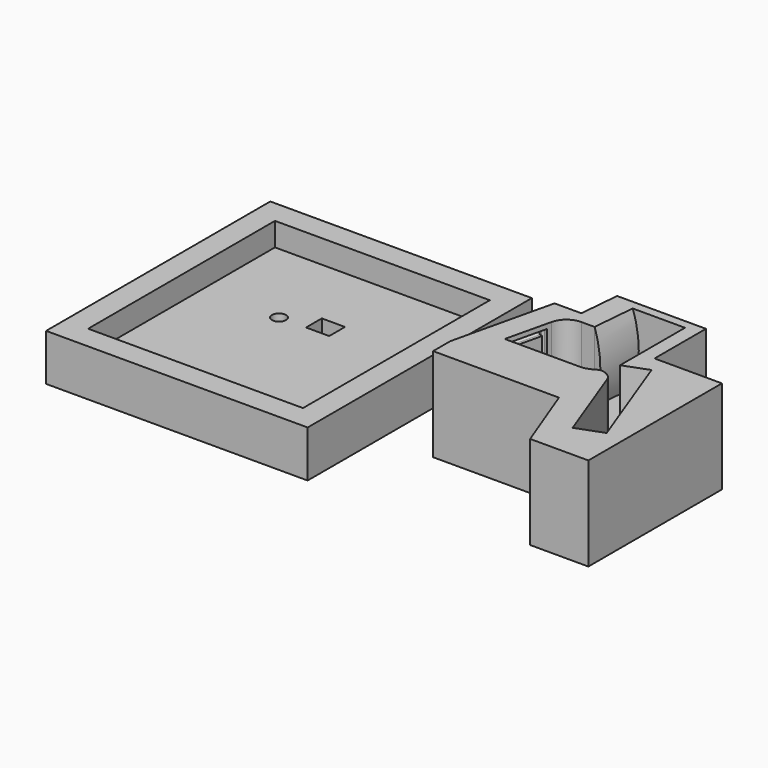
from build123d import *

# Parameters (mm, degrees)
F1_DEPTH      = 15
F4_DEPTH      = 9.2
F4_DEPTH_BACK = 1
F6_R          = 1.5
F7_DEPTH      = 20
F9_R          = 1.5
F10_DEPTH     = 5
F11_W         = 56
F11_H         = 60
F11_R         = 1.5
F11_W_2       = 4.962
F11_H_2       = 4.2207975686
F12_DEPTH     = 5
F14_W         = 56
F14_H         = 60
F14_W_2       = 46
F14_H_2       = 50
F15_DEPTH     = 5
F20_W         = 7.9759681362
F20_H         = 13
F20_W_2       = 5.9759681362
F20_H_2       = 11
F21_DEPTH     = 1
F22_R         = 0.4


# Not quite as in the source:
# - the program builds the solid bodies; features that only make, move or delete a surface that nothing else refers to are left out


with BuildPart() as f1:
    # F0 (on Top) → F1 (new body)
    with BuildSketch(Plane.XY):
        with BuildLine():
            Line((2.2764293651, 9.7127652912), (0, 0))
            Line((0, 0), (16, 0))
            ThreePointArc((16, 0), (17.4448615439, 0.2133127198), (18.7664401496, 0.8350499525))
            ThreePointArc((18.7664401496, 0.8350499525), (19.8489592754, 1.1689252442), (20.9391965895, 0.8611867726))
            ThreePointArc((20.9391965895, 0.8611867726), (21.8699515292, 0.2737220948), (22.4677167157, -0.6504512046))
            Line((22.4677167157, -0.6504512046), (28.953752481, -18.0237612902))
            Line((28.953752481, -18.0237612902), (34.5748015694, -15.9252362972))
            Line((34.5748015694, -15.9252362972), (26.1807015974, 6.5589600562))
            Line((26.1807015974, 6.5589600562), (21, 4.6248314599))
            Line((21, 4.6248314599), (21, 22))
            Line((21, 22), (9.8, 22))
            Line((9.8, 22), (9.0007942351, 12.8091337038))
            ThreePointArc((9.0007942351, 12.8091337038), (8.9975896779, 12.8026290109), (8.9908318292, 12.8))
            Line((8.9908318292, 12.8), (6.1708946074, 12.8))
            ThreePointArc((6.1708946074, 12.8), (3.6860466407, 11.9345702389), (2.2764293651, 9.7127652912))
        make_face()
    extrude(amount=F1_DEPTH)

    # F3 (on face) → F4 (cut, two sides)
    with BuildSketch(Plane(origin=(1.9722326454, 22.6806754221, 0), x_dir=(0.9962405882, -0.0866296164, 0), z_dir=(-0.0866296164, -0.9962405882, 0))) as f4_sk:
        with BuildLine():
            Line((7.8573062043, 15), (7.8573062043, 0))
            ThreePointArc((7.8573062043, 0), (9.161162664, 7.5), (7.8573062043, 15))
        make_face()
    extrude(amount=F4_DEPTH, mode=Mode.SUBTRACT)
    extrude(f4_sk.sketch, amount=-F4_DEPTH_BACK, mode=Mode.SUBTRACT)


with BuildPart() as f7:
    # F6 (on offset) → F7 (new body)
    with BuildSketch(Plane.XY.offset(-5)):
        Polygon((23.9650979638, 23.9009789079), (4.9464345222, 23.9009789079), (4.1964484146, 15.2761386707), (-1.5551482583, 15.2761386707), (-6.6067720969, -6.2774563741), (-6.6067720969, -10.9053393826), (20.3434042633, -10.9053393826), (25.9253627227, -25.5990210921), (38.3932279031, -25.5990210921), (38.3932279031, 10.140940547), (23.9650979638, 10.140940547), align=None)
        with Locations((16, 5)):
            Circle(F6_R, mode=Mode.SUBTRACT)
    extrude(amount=F7_DEPTH)

    # F8: cut F1
    add(f1.part, mode=Mode.SUBTRACT)

    # F9 (on offset) → F10 (cut)
    with BuildSketch(Plane.XY.offset(-5)):
        with Locations((16, 5)):
            Circle(F9_R)
    extrude(amount=F10_DEPTH, mode=Mode.SUBTRACT)

    # F20 (on offset) → F21 (cut)
    with BuildSketch(Plane(origin=(0, 0, 0), x_dir=(0.2281913228, 0.9736163106, 0), z_dir=(0.9736163106, -0.2281913228, 0))):
        with Locations((4.9879840681, 7.5)):
            Rectangle(F20_W, F20_H)
        with Locations((4.9879840681, 7.5)):
            Rectangle(F20_W_2, F20_H_2, mode=Mode.SUBTRACT)
    extrude(amount=-F21_DEPTH, mode=Mode.SUBTRACT)

    # F22
    f22_edges = [f7.edges().sort_by_distance(p)[0] for p in [
        (1.074622, 8.96734, 7.5),
        (0.164598, 5.084574, 14),
        (-0.745425, 1.201808, 7.5),
        (0.164598, 5.084574, 1),
        (0.84643, 7.993724, 7.5),
        (0.164598, 5.084574, 13),
        (-0.517234, 2.175424, 7.5),
        (0.164598, 5.084574, 2),
    ]]
    fillet(f22_edges, radius=F22_R)


with BuildPart() as f12:
    # F11 (on offset) → F12 (new body)
    with BuildSketch(Plane.XY.offset(-5)):
        with Locations((-45.7067461014, -0.5990204215)):
            Rectangle(F11_W, F11_H)
        with Locations((-52.3137461014, 5)):
            Circle(F11_R, mode=Mode.SUBTRACT)
        with Locations((-44.052677727, 7.1103987843)):
            Rectangle(F11_W_2, F11_H_2, mode=Mode.SUBTRACT)
    extrude(amount=F12_DEPTH)

    # F14 (on offset) → F15 (join)
    with BuildSketch(Plane.XY):
        with Locations((-45.7067461014, -0.5990204215)):
            Rectangle(F14_W, F14_H)
        with Locations((-45.7067461014, -0.5990204215)):
            Rectangle(F14_W_2, F14_H_2, mode=Mode.SUBTRACT)
    extrude(amount=F15_DEPTH)


solid = Compound([f7.part, f12.part])
